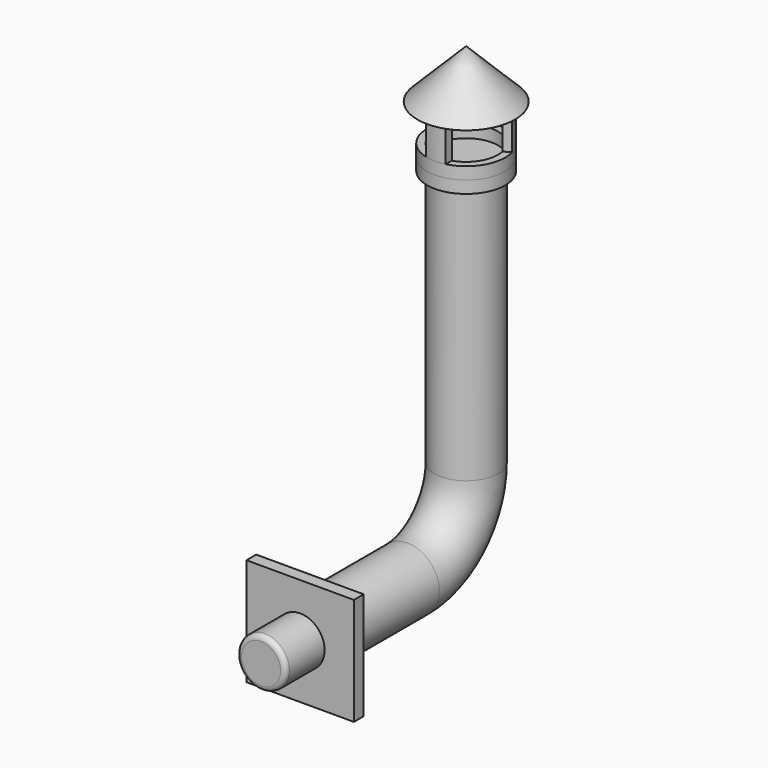
from build123d import *

# Parameters (mm, degrees)
F1_R             = 1.3
F3_W             = 4.4
F3_H             = 4.4
F3_R             = 1.3
F4_DEPTH         = 0.5
F5_R             = 1
F6_DEPTH         = 2
F7_R             = 0.2
F8_R             = 1.6
F8_R_2           = 1.3
F9_DEPTH         = 0.5
F9_DEPTH_BACK    = 0.5
F11_DEPTH        = 1.5
F11_COPIES_COUNT = 3


# Not quite as in the source:
# - a pattern or mirror of a feature is missing from the dataset's text; its kind, count and spacing are read off the source's solid


with BuildPart() as f2:
    # F2: sweep along a path in F0
    with BuildLine(Plane.YZ) as f2_path:
        Line((0, 0), (5, 0))
        ThreePointArc((5, 0), (7.1213203436, 0.8786796564), (8, 3))
        Line((8, 3), (8, 14))
    # F1 (on Front) → F2 (sweep)
    with BuildSketch(Plane.XZ):
        Circle(F1_R)
    sweep(path=f2_path.line)

    # F3 (on face) → F4 (join)
    with BuildSketch(Plane.XZ):
        Rectangle(F3_W, F3_H)
        Circle(F3_R, mode=Mode.SUBTRACT)
        Circle(F3_R)
    extrude(amount=F4_DEPTH)

    # F5 (on face) → F6 (join)
    with BuildSketch(Plane.XZ.offset(0.5)):
        Circle(F5_R)
    extrude(amount=F6_DEPTH)

    # F7
    f7_edges = [f2.edges().sort_by_distance(p)[0] for p in [
        (-1, -2.5, 0),
    ]]
    fillet(f7_edges, radius=F7_R)

    # F8 (on face) → F9 (join, two sides)
    with BuildSketch(Plane.XY.offset(14)) as f9_sk:
        with Locations((0, 8)):
            Circle(F8_R)
        with Locations((0, 8)):
            Circle(F8_R_2, mode=Mode.SUBTRACT)
    extrude(amount=-F9_DEPTH)
    extrude(f9_sk.sketch, amount=F9_DEPTH_BACK)

    # F10 (on face) → F11 (join)
    with BuildSketch(Plane.XY.offset(14.5)):
        with BuildLine():
            Line((-0.4, 6.7630683123), (-0.4, 6.4508066615))
            ThreePointArc((-0.4, 6.4508066615), (0, 6.4), (0.4, 6.4508066615))
            Line((0.4, 6.4508066615), (0.4, 6.7630683123))
            ThreePointArc((0.4, 6.7630683123), (0, 6.7), (-0.4, 6.7630683123))
        make_face()
    f11 = extrude(amount=F11_DEPTH)

    # F11_copies: F11 ×3 about axis
    f11_copies_axis = Axis((0, 8, 0), (0, 0, 1))
    for i in range(1, F11_COPIES_COUNT):
        add(f11.rotate(f11_copies_axis, i * 360 / F11_COPIES_COUNT))

    # F13 (on Right) → F14 (revolve)
    with BuildSketch(Plane.YZ):
        Polygon((6, 16), (6.4508066615, 16), (6.7630683123, 16), (8, 16), (8, 18), align=None)
    revolve(axis=Axis((0, 8, 17.9220158607), (0, 0, 1)))


solid = f2.part
